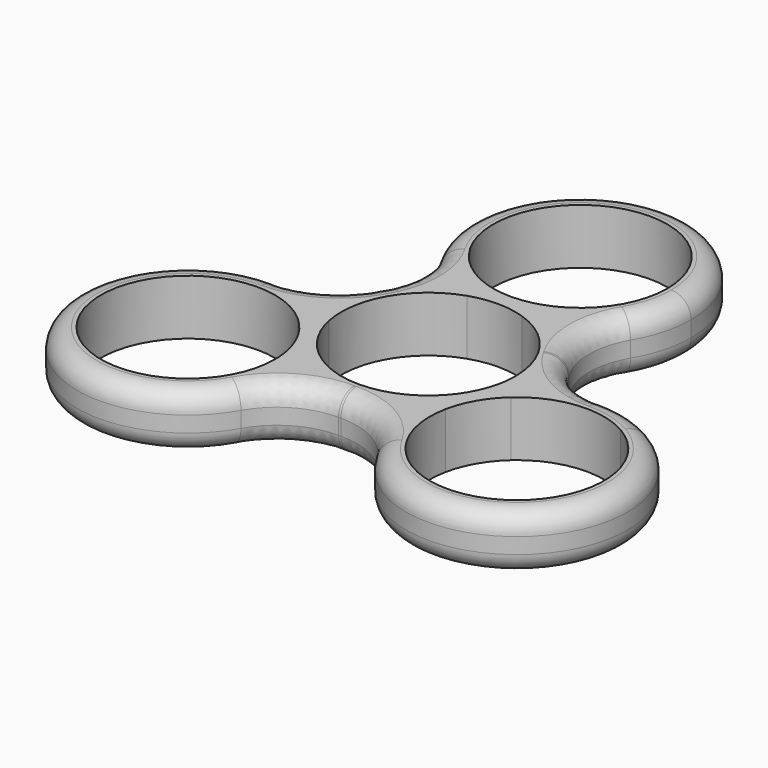
from build123d import *

# Parameters (mm, degrees)
F1_DEPTH = 7
F2_R     = 9.5597147321
F3_R     = 2.5


# Not quite as in the source:
# - a pattern or mirror of a feature is missing from the dataset's text; its kind, count and spacing are read off the source's solid


with BuildPart() as f1:
    # F0 (on Top) → F1 (new body)
    with BuildSketch(Plane.XY):
        with BuildLine():
            ThreePointArc((3.4725485958, 13.5625), (5.3986527966, 12.9172190498), (7.2111025509, 12))
            ThreePointArc((7.2111025509, 12), (12.1851433252, 17.1063592969), (14, 24))
            ThreePointArc((14, 24), (-6.8936407031, 36.1851433252), (-7.2111025509, 12))
            ThreePointArc((-7.2111025509, 12), (-5.3986527966, 12.9172190498), (-3.4725485958, 13.5625))
            ThreePointArc((-3.4725485958, 13.5625), (-6.4343595426, 32.9218281354), (11, 24))
            ThreePointArc((11, 24), (8.9218281354, 17.5656404574), (3.4725485958, 13.5625))
        make_face()
        with BuildLine():
            ThreePointArc((-10.7754144499, -2.2114347002), (-9.5262794416, 5.5), (-3.4725485958, 10.4375))
            ThreePointArc((-3.4725485958, 10.4375), (-5.3986527966, 11.0827809502), (-7.2111025509, 12))
            ThreePointArc((-7.2111025509, 12), (-12.124355653, 7), (-13.9978561209, 0.2449979984))
            ThreePointArc((-13.9978561209, 0.2449979984), (-12.2972962457, -0.866020007), (-10.7754144499, -2.2114347002))
        make_face()
        with BuildLine():
            ThreePointArc((-13.4817438367, -3.7739347002), (-13.8859662417, -1.7832390568), (-13.9978561209, 0.2449979984))
            ThreePointArc((-13.9978561209, 0.2449979984), (-32.9089653438, -19), (-6.7867535699, -12.2449979984))
            ThreePointArc((-6.7867535699, -12.2449979984), (-8.4873134451, -11.133979993), (-10.0091952409, -9.7885652998))
            ThreePointArc((-10.0091952409, -9.7885652998), (-9.8409001061, -10.8885952467), (-9.7846096908, -12))
            ThreePointArc((-9.7846096908, -12), (-30.8178425795, -16.5093500421), (-13.4817438367, -3.7739347002))
        make_face()
        with BuildLine():
            ThreePointArc((-7.3028658541, -8.2260652998), (-9.5262794416, -5.5), (-10.7754144499, -2.2114347002))
            ThreePointArc((-10.7754144499, -2.2114347002), (-12.2972962457, -0.866020007), (-13.9978561209, 0.2449979984))
            ThreePointArc((-13.9978561209, 0.2449979984), (-13.8859662417, -1.7832390568), (-13.4817438367, -3.7739347002))
            ThreePointArc((-13.4817438367, -3.7739347002), (-11.2583302492, -6.5), (-10.0091952409, -9.7885652998))
            ThreePointArc((-10.0091952409, -9.7885652998), (-8.4873134451, -11.133979993), (-6.7867535699, -12.2449979984))
            ThreePointArc((-6.7867535699, -12.2449979984), (-6.7851456709, -12.1225036892), (-6.7846096908, -12))
            ThreePointArc((-6.7846096908, -12), (-6.9147788751, -10.0953233495), (-7.3028658541, -8.2260652998))
        make_face()
        with BuildLine():
            ThreePointArc((13.9978561209, 0.2449979984), (12.2972962457, -0.866020007), (10.7754144499, -2.2114347002))
            ThreePointArc((10.7754144499, -2.2114347002), (9.5262794416, -5.5), (7.3028658541, -8.2260652998))
            ThreePointArc((7.3028658541, -8.2260652998), (6.8986434491, -10.2167609432), (6.7867535699, -12.2449979984))
            ThreePointArc((6.7867535699, -12.2449979984), (8.4873134451, -11.133979993), (10.0091952409, -9.7885652998))
            ThreePointArc((10.0091952409, -9.7885652998), (11.2583302492, -6.5), (13.4817438367, -3.7739347002))
            ThreePointArc((13.4817438367, -3.7739347002), (13.8698308157, -1.9046766505), (14, 0))
            ThreePointArc((14, 0), (13.99946402, 0.1225036892), (13.9978561209, 0.2449979984))
        make_face()
        with BuildLine():
            ThreePointArc((6.7867535699, -12.2449979984), (6.8986434491, -10.2167609432), (7.3028658541, -8.2260652998))
            ThreePointArc((7.3028658541, -8.2260652998), (0, -11), (-7.3028658541, -8.2260652998))
            ThreePointArc((-7.3028658541, -8.2260652998), (-6.9147788751, -10.0953233495), (-6.7846096908, -12))
            ThreePointArc((-6.7846096908, -12), (-6.7851456709, -12.1225036892), (-6.7867535699, -12.2449979984))
            ThreePointArc((-6.7867535699, -12.2449979984), (0, -14), (6.7867535699, -12.2449979984))
        make_face()
        with BuildLine():
            ThreePointArc((3.4725485958, 10.4375), (8.9218281354, 6.4343595426), (11, 0))
            ThreePointArc((11, 0), (10.9437095847, -1.1114047533), (10.7754144499, -2.2114347002))
            ThreePointArc((10.7754144499, -2.2114347002), (12.2972962457, -0.866020007), (13.9978561209, 0.2449979984))
            ThreePointArc((13.9978561209, 0.2449979984), (12.124355653, 7), (7.2111025509, 12))
            ThreePointArc((7.2111025509, 12), (5.3986527966, 11.0827809502), (3.4725485958, 10.4375))
        make_face()
        with BuildLine():
            ThreePointArc((-3.4725485958, 10.4375), (0, 11), (3.4725485958, 10.4375))
            ThreePointArc((3.4725485958, 10.4375), (5.3986527966, 11.0827809502), (7.2111025509, 12))
            ThreePointArc((7.2111025509, 12), (5.3986527966, 12.9172190498), (3.4725485958, 13.5625))
            ThreePointArc((3.4725485958, 13.5625), (0, 13), (-3.4725485958, 13.5625))
            ThreePointArc((-3.4725485958, 13.5625), (-5.3986527966, 12.9172190498), (-7.2111025509, 12))
            ThreePointArc((-7.2111025509, 12), (-5.3986527966, 11.0827809502), (-3.4725485958, 10.4375))
        make_face()
    extrude(amount=F1_DEPTH)

    # F1_copies: F1 across plane


with BuildPart() as f1_1:
    add(f1.part)
    add(f1.part.mirror(Plane(origin=(0, 0, 0), x_dir=(-0.8660254038, -0.5, 0), z_dir=(0.5, -0.8660254038, 0))))

    # F2
    f2_edges = [f1_1.edges().sort_by_distance(p)[0] for p in [
        (7.211103, 12, 3.5),
        (13.997856, 0.244998, 3.5),
        (-13.997856, 0.244998, 3.5),
        (-7.211103, 12, 3.5),
        (-6.786754, -12.244998, 3.5),
        (6.786754, -12.244998, 3.5),
    ]]
    fillet(f2_edges, radius=F2_R)

    # F3
    f3_edges = [f1_1.edges().sort_by_distance(p)[0] for p in [
        (-32.908965, -19, 7),
        (32.908965, -19, 7),
        (0, 38, 7),
        (0, 38, 0),
        (-10.714904, 12, 0),
        (-32.908965, -19, 0),
        (32.908965, -19, 0),
        (10.714904, 12, 0),
        (12.124356, 7, 0),
        (-12.124356, 7, 0),
        (15.749757, 3.279379, 0),
        (-15.749757, 3.279379, 0),
        (5.034853, -15.279379, 0),
        (-5.034853, -15.279379, 0),
        (0, -14, 0),
        (10.714904, 12, 7),
        (-10.714904, 12, 7),
        (12.124356, 7, 7),
        (-12.124356, 7, 7),
        (15.749757, 3.279379, 7),
        (-15.749757, 3.279379, 7),
        (5.034853, -15.279379, 7),
        (-5.034853, -15.279379, 7),
        (0, -14, 7),
    ]]
    fillet(f3_edges, radius=F3_R)


solid = f1_1.part
